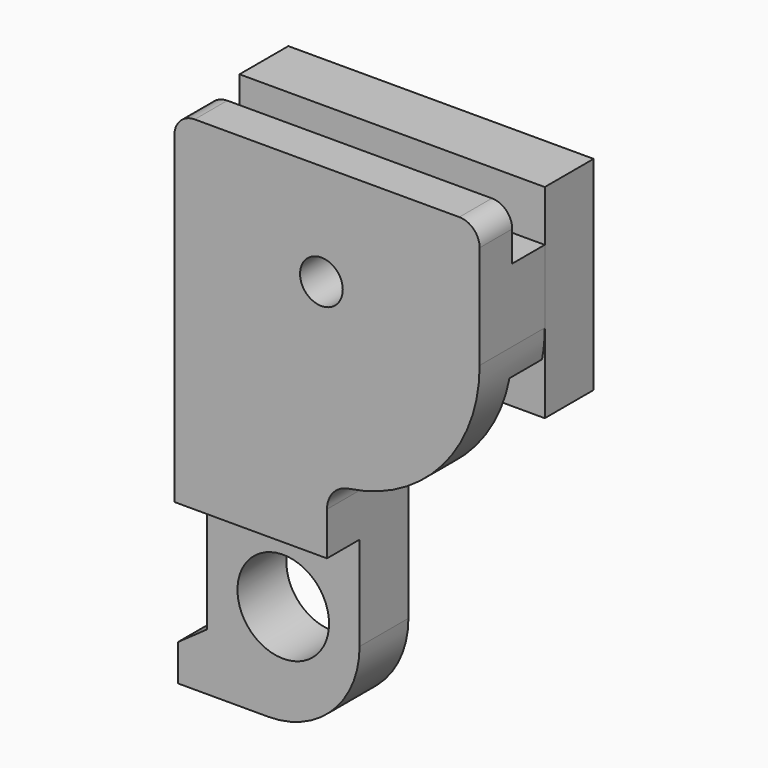
from build123d import *

# Parameters (mm, degrees)
F0_W        = 30
F0_H        = 5
F0_R        = 2.1
F0_W_2      = 15
F0_H_2      = 6.75205
F1_DEPTH    = 4
F2_DEPTH    = 4
F3_DEPTH    = 6
F4_DEPTH    = 5
F0_R_2      = 4.5
F5_DEPTH    = 6
F6_DEPTH    = 5
F7_R        = 2.5
F8_T1_DEPTH = 78.1025403784
F9_DEPTH    = 6
F10_R       = 9
F11_R       = 2


# Not quite as in the source:
# - a fillet or chamfer that OpenCascade refuses, or shapes differently, is made with other operations: its cross-section is extruded or revolved along the edge and cut away or added


with BuildPart() as f1:
    # F0 (on Front) → F1 (new body)
    with BuildSketch(Plane.XZ):
        with Locations((-7.0197439194, 16.2580000609)):
            Rectangle(F0_W, F0_H)
        Polygon((7.9802560806, 13.7580000609), (-22.0197439194, 13.7580000609), (-22.0197439194, 3.7580000609), (-7.0197439194, 3.7580000609), (7.9802560806, 3.7580000609), align=None)
        with Locations((-7.5721158646, 8.7580000609)):
            Circle(F0_R, mode=Mode.SUBTRACT)
        Polygon((-7.0197439194, 3.7580000609), (-22.0197439194, 3.7580000609), (-22.0197439194, -8.2419999391), (-7.0197439194, -8.2419999391), (7.9802560806, -8.2419999391), (7.9802560806, 3.7580000609), align=None)
        with Locations((-14.5197439194, -11.6180249391)):
            Rectangle(F0_W_2, F0_H_2)
    extrude(amount=F1_DEPTH)

    # F0 (on Front) → F2 (join)
    with BuildSketch(Plane.XZ):
        Polygon((7.9802560806, 13.7580000609), (-22.0197439194, 13.7580000609), (-22.0197439194, 3.7580000609), (-7.0197439194, 3.7580000609), (7.9802560806, 3.7580000609), align=None)
        with Locations((-7.5721158646, 8.7580000609)):
            Circle(F0_R, mode=Mode.SUBTRACT)
    extrude(amount=-F2_DEPTH)


with BuildPart() as f3:
    # F3 (new): a face of the model
    f3_faces = [f1.part.faces().sort_by_distance(p)[0] for p in [
        (-7.0197439194, 4, 13.4417722949),
    ]]
    extrude(f3_faces, amount=F3_DEPTH)

    # F4 (add): a face of the model
    f4_faces = [f3.faces().sort_by_distance(p)[0] for p in [
        (-7.0197439194, 7, 3.7580000609),
    ]]
    extrude(f4_faces, amount=F4_DEPTH)

    # F6 (add): a face of the model
    f6_faces = [f3.faces().sort_by_distance(p)[0] for p in [
        (-7.0197439194, 7, 13.7580000609),
    ]]
    extrude(f6_faces, amount=F6_DEPTH)


with BuildPart() as f1_1:
    add(f1.part)

    # F0 (on Front) → F5 (join)
    with BuildSketch(Plane.XZ):
        with Locations((-14.5197439194, -11.6180249391)):
            Rectangle(F0_W_2, F0_H_2)
        Polygon((-7.0197439194, -14.9940499391), (-22.0197439194, -14.9940499391), (-22.0197439194, -27.6507474482), (-22.0197439194, -33.2419999391), (-7.0197439194, -33.2419999391), align=None)
        with Locations((-14.5197439194, -23.2419999391)):
            Circle(F0_R_2, mode=Mode.SUBTRACT)
    extrude(amount=-F5_DEPTH)

    # F7
    f7_edges = [f1_1.edges().sort_by_distance(p)[0] for p in [
        (-7.019744, -2, -8.242),
    ]]
    fillet(f7_edges, radius=F7_R)

    # F8: fillet of radius 15 on 1 edges, made by hand

    # F8_s2 → F8_t1 (cut)
    with BuildSketch(Plane.XZ.offset(-37.0512701892)):
        with BuildLine():
            ThreePointArc((-4.8768867765, -8.2676416426), (4.3191902709, -3.241296924), (7.9802560806, 6.5785081366))
            Line((7.9802560806, 6.5785081366), (9.4802560806, 6.5785081366))
            Line((9.4802560806, 6.5785081366), (9.4802560806, -8.2419999391))
            Line((9.4802560806, -8.2419999391), (7.9802560806, -9.7419999391))
            ThreePointArc((7.9802560806, -9.7419999391), (-4.5197439194, -9.7419999391), (-4.6626010622, -9.7522566205))
            Line((-4.6626010622, -9.7522566205), (-4.8768867765, -8.2676416426))
        make_face()
    extrude(amount=F8_T1_DEPTH, mode=Mode.SUBTRACT)

    # F0 (on Front) → F9 (join)
    with BuildSketch(Plane.XZ):
        Polygon((-22.0197439194, -33.2419999391), (-22.0197439194, -27.6507474482), (-24.877268821, -29.6678245068), (-24.877268821, -33.2419999391), align=None)
    extrude(amount=-F9_DEPTH)

    # F10
    f10_edges = [f1_1.edges().sort_by_distance(p)[0] for p in [
        (-7.019744, 3, -33.242),
    ]]
    fillet(f10_edges, radius=F10_R)

    # F11
    f11_edges = [f1_1.edges().sort_by_distance(p)[0] for p in [
        (-22.019744, -2, 18.758),
        (7.980256, -2, 18.758),
    ]]
    fillet(f11_edges, radius=F11_R)


solid = Compound([f3.part, f1_1.part])
